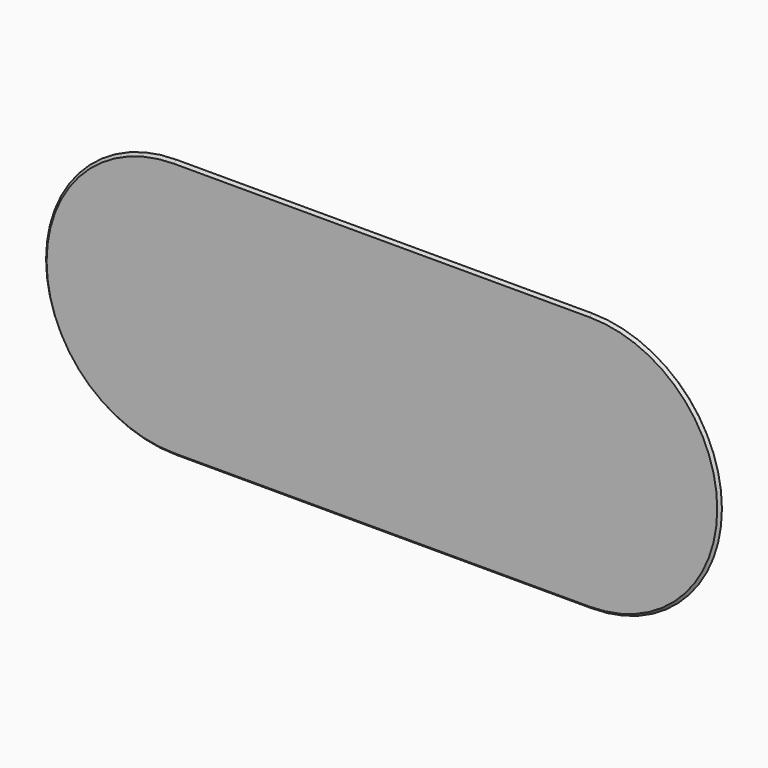
from build123d import *

# Parameters (mm, degrees)
F1_DEPTH = 1
F2_SIZE  = 0.49999


# Not quite as in the source:
# - a fillet or chamfer is up to 0.001 mm smaller than in the source, because OpenCascade refuses the exact size


with BuildPart() as f1:
    # F0 (on Front) → F1 (new body)
    with BuildSketch(Plane.XZ):
        with BuildLine():
            ThreePointArc((40, -25), (65, 0), (40, 25))
            Line((40, 25), (-40, 25))
            ThreePointArc((-40, 25), (-65, 0), (-40, -25))
            Line((-40, -25), (40, -25))
        make_face()
    extrude(amount=F1_DEPTH)

    # F2 (size 0.5 in the source; OpenCascade refuses exactly that, so slightly less here)
    f2_edges = [f1.edges().sort_by_distance(p)[0] for p in [
        (0, -1, 25),
        (0, 0, 25),
    ]]
    chamfer(f2_edges, length=F2_SIZE)


solid = f1.part
